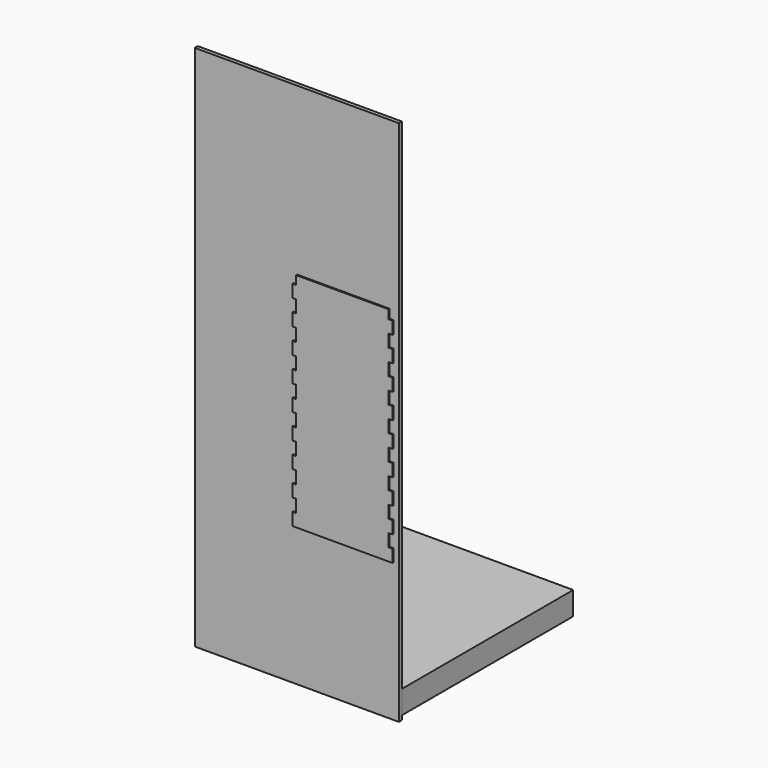
from build123d import *

# Parameters (mm, degrees)
F0_W     = 162.62761
F0_H     = 420
F1_DEPTH = 3
F2_W     = 170.722424984
F2_H     = 18.5404643416
F3_DEPTH = 118.454916951
F4_DEPTH = 44.172693049
F6_DEPTH = 4


# Not quite as in the source:
# - a feature of the source that left no trace in its solid (it failed there, or was rolled back) is left out


with BuildPart() as f1:
    # F0 (on Front) → F1 (new body)
    with BuildSketch(Plane.XZ):
        with Locations((-37.141111951, 5.6345053017)):
            Rectangle(F0_W, F0_H)
    extrude(amount=F1_DEPTH)


with BuildPart() as f3:
    # F2 (on Right) → F3 (new body, through all)
    with BuildSketch(Plane.YZ):
        with Locations((85.361212492, -191.6734613478)):
            Rectangle(F2_W, F2_H)
    extrude(amount=-F3_DEPTH)

    # F4 (add, through all): a face of the model
    f4_faces = [f3.faces().sort_by_distance(p)[0] for p in [
        (0, 85.361212492, -191.6734613478),
    ]]
    extrude(f4_faces, amount=F4_DEPTH)


with BuildPart() as f6:
    # F5 (on Front) → F6 (new body)
    with BuildSketch(Plane.XZ):
        Polygon((-39.788750782, -83.8537883393), (-39.788750782, -93.8537883393), (39.788750782, -93.8537883393), (39.788750782, -83.8537883393), (36.788750782, -83.8537883393), (36.788750782, -73.8537883393), (39.788750782, -73.8537883393), (39.788750782, -63.8537883393), (36.788750782, -63.8537883393), (36.788750782, -53.8537883393), (39.788750782, -53.8537883393), (39.788750782, -43.8537883393), (36.788750782, -43.8537883393), (36.788750782, -33.8537883393), (39.788750782, -33.8537883393), (39.788750782, -23.8537883393), (36.788750782, -23.8537883393), (36.788750782, -13.8537883393), (39.788750782, -13.8537883393), (39.788750782, -3.8537883393), (36.788750782, -3.8537883393), (36.788750782, 6.1462116607), (39.788750782, 6.1462116607), (39.788750782, 16.1462116607), (36.788750782, 16.1462116607), (36.788750782, 26.1462116607), (39.788750782, 26.1462116607), (39.788750782, 36.1462116607), (36.788750782, 36.1462116607), (36.788750782, 46.1462116607), (39.788750782, 46.1462116607), (39.788750782, 56.1462116607), (36.788750782, 56.1462116607), (36.788750782, 66.1462116607), (39.788750782, 66.1462116607), (39.788750782, 76.1462116607), (36.788750782, 76.1462116607), (36.788750782, 83.0940887698), (-36.788750782, 83.0940887698), (-36.788750782, 76.1462116607), (-39.788750782, 76.1462116607), (-39.788750782, 66.1462116607), (-36.788750782, 66.1462116607), (-36.788750782, 56.1462116607), (-39.788750782, 56.1462116607), (-39.788750782, 46.1462116607), (-36.788750782, 46.1462116607), (-36.788750782, 36.1462116607), (-39.788750782, 36.1462116607), (-39.788750782, 26.1462116607), (-36.788750782, 26.1462116607), (-36.788750782, 16.1462116607), (-39.788750782, 16.1462116607), (-39.788750782, 6.1462116607), (-36.788750782, 6.1462116607), (-36.788750782, -3.8537883393), (-39.788750782, -3.8537883393), (-39.788750782, -13.8537883393), (-36.788750782, -13.8537883393), (-36.788750782, -23.8537883393), (-39.788750782, -23.8537883393), (-39.788750782, -33.8537883393), (-36.788750782, -33.8537883393), (-36.788750782, -43.8537883393), (-39.788750782, -43.8537883393), (-39.788750782, -53.8537883393), (-36.788750782, -53.8537883393), (-36.788750782, -63.8537883393), (-39.788750782, -63.8537883393), (-39.788750782, -73.8537883393), (-36.788750782, -73.8537883393), (-36.788750782, -83.8537883393), align=None)
    extrude(amount=F6_DEPTH)


solid = Compound([f1.part, f3.part, f6.part])
